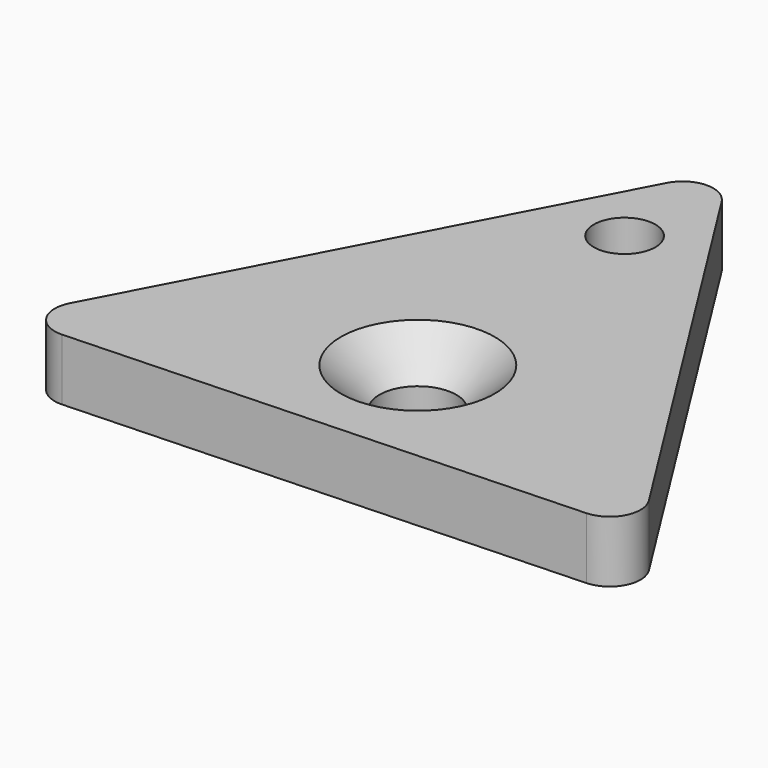
from build123d import *

# Parameters (mm, degrees)
F0_R           = 1
F1_DEPTH       = 2
F3_D           = 2.5
F3_DEPTH       = 15.81
F3_CSINK_D     = 5
F3_CSINK_ANGLE = 90
F3_TIP         = 0.7510757738


# Not quite as in the source:
# - a feature names something its author has since deleted; it is built from what else it names


with BuildPart() as f1:
    # F0 (on Top) → F1 (new body)
    with BuildSketch(Plane.XY):
        with BuildLine():
            Line((-8.0353952667, -6.0930074749), (8.4878063746, -5.4451317825))
            ThreePointArc((8.4878063746, -5.4451317825), (9.3335768433, -4.9115848639), (9.2943968921, -3.912352693))
            Line((9.2943968921, -3.912352693), (0.4717192633, 10.0732218341))
            ThreePointArc((0.4717192633, 10.0732218341), (-0.4132311567, 10.5389070865), (-1.2590016254, 10.0053601679))
            Line((-1.2590016254, 10.0053601679), (-8.9595256379, -4.6280900516))
            ThreePointArc((-8.9595256379, -4.6280900516), (-8.9203456867, -5.6273222225), (-8.0353952667, -6.0930074749))
        make_face()
        with Locations((-0.2769940404, 7.0643619393)):
            Circle(F0_R, mode=Mode.SUBTRACT)
    extrude(amount=F1_DEPTH)

    # F3
    with Locations(Plane.XY.offset(2)):
        with Locations((0.0693653225, -1.7690696287)):
            CounterSinkHole(F3_D / 2, F3_CSINK_D / 2, depth=F3_DEPTH, counter_sink_angle=F3_CSINK_ANGLE)
            with Locations((0, 0, -(F3_DEPTH + F3_TIP / 2))):  # 118° drill point
                Cone(0, F3_D / 2, F3_TIP, mode=Mode.SUBTRACT)


solid = f1.part
